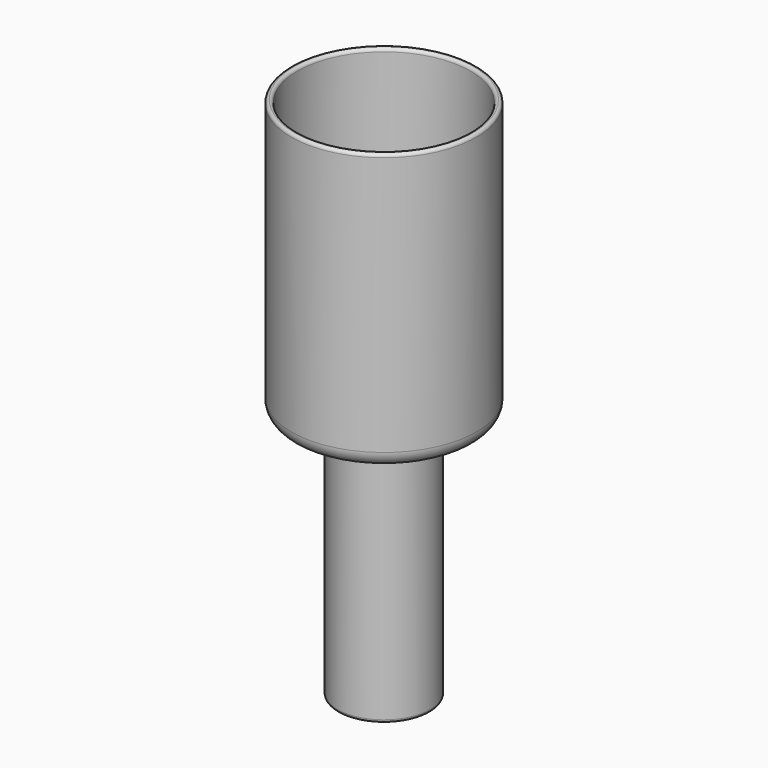
from build123d import *

# Parameters (mm, degrees)
F2_R = 5
F3_R = 0.99999


# Not quite as in the source:
# - a fillet or chamfer is up to 0.001 mm smaller than in the source, because OpenCascade refuses the exact size


with BuildPart() as f1:
    # F0 (on Front) → F1 (revolve)
    with BuildSketch(Plane.XZ):
        Polygon((-28, 10.3754994379), (-28, 98.3754994379), (-30, 98.3754994379), (-30, 8.3754994379), (-15, 8.3754994379), (-15, -71.6245005621), (-13, -71.6245005621), (-13, 10.3754994379), align=None)
    revolve(axis=Axis((0, 0, 13.3754994379), (0, 0, -1)))

    # F2
    f2_edges = [f1.edges().sort_by_distance(p)[0] for p in [
        (30, 0, 8.375499),
        (15, 0, 8.375499),
        (28, 0, 10.375499),
        (13, 0, 10.375499),
    ]]
    fillet(f2_edges, radius=F2_R)

    # F3 (radius 1 in the source; OpenCascade refuses exactly that, so slightly less here)
    f3_edges = [f1.edges().sort_by_distance(p)[0] for p in [
        (28, 0, 98.375499),
        (30, 0, 98.375499),
        (15, 0, -71.624501),
        (13, 0, -71.624501),
    ]]
    fillet(f3_edges, radius=F3_R)


solid = f1.part
